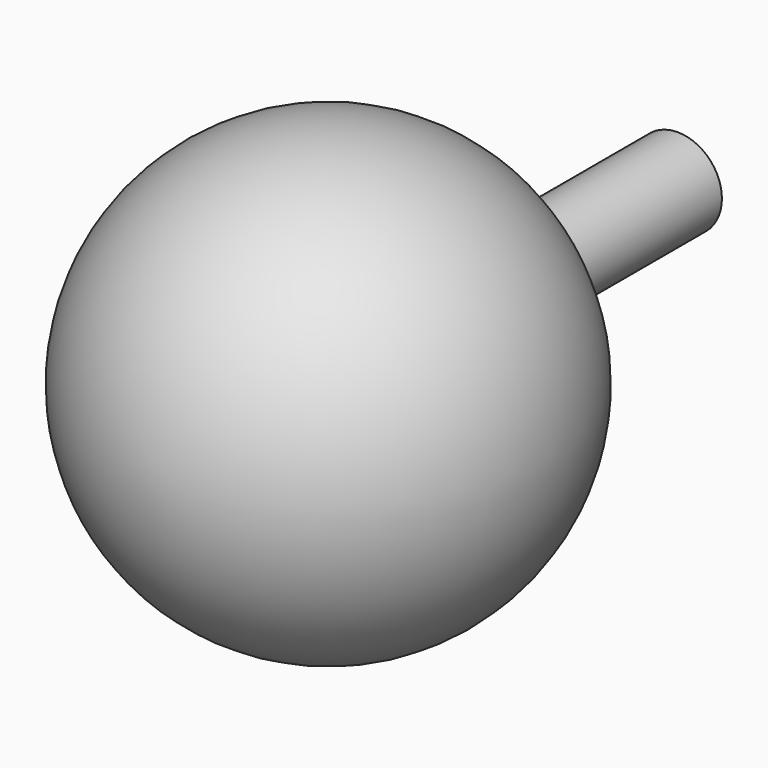
from build123d import *


# Not quite as in the source:
# - a feature names something its author has since deleted; it is built from what else it names


with BuildPart() as f1:
    # F0 (on Top) → F1 (revolve)
    with BuildSketch(Plane.XY):
        with BuildLine():
            Line((0, 9.7979589711), (0, -10))
            ThreePointArc((0, -10), (9.9493615301, -1.0050896201), (2, 9.7979589711))
            Line((2, 9.7979589711), (2, 19.7979589711))
            Line((2, 19.7979589711), (0, 19.7979589711))
            Line((0, 19.7979589711), (0, 9.7979589711))
        make_face()
    revolve(axis=Axis((0, -0.1010205144, 0), (0, -1, 0)))


solid = f1.part
